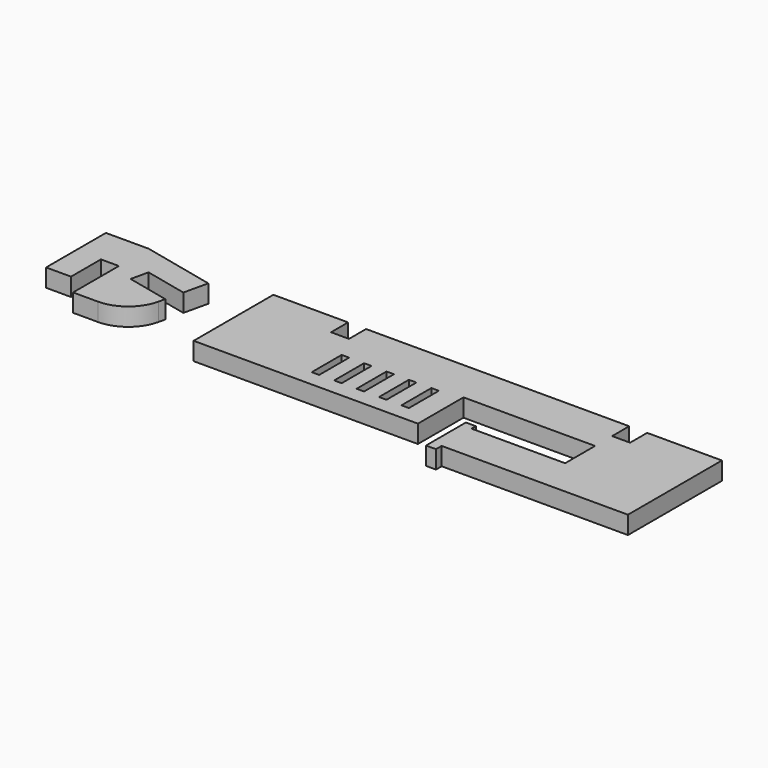
from build123d import *

# Parameters (mm, degrees)
F1_W     = 25.4
F1_H     = 38.1
F2_DEPTH = 18.288
F1_W_2   = 7.62
F1_W_3   = 95.377
F1_H_2   = 18.1300078465
F1_H_3   = 19.9699921535
F1_W_4   = 76.2


# Not quite as in the source:
# - a variable given as a bare number and used for a length is read in inches; the dataset says mm whatever the document's units were


with BuildPart() as f2:
    # F1 (on Top) → F2 (new body)
    with BuildSketch(Plane.XY):
        Polygon((-25.4, 57.9158396344), (-25.4, 19.8158396344), (-25.4, 5.8057135582), (0, 0), (37.5647200947, -8.58622066), (39.1494498942, -1.6530269181), (-4.1830109925, 8.2515343291), (-0.1079915079, 26.0797468083), (43.2244693788, 16.175185561), (48.884218663, 40.936591782), align=None)
        with BuildLine():
            Line((37.5647200947, -8.58622066), (0, 0))
            Line((0, 0), (0, -38.5335098455))
            ThreePointArc((0, -38.5335098455), (24.020555392, -30.1304546875), (37.5647200947, -8.58622066))
        make_face()
        Polygon((-69.088, 19.8158396344), (-43.688, 19.8158396344), (-25.4, 19.8158396344), (-25.4, 57.9158396344), (-69.088, 57.9158396344), align=None)
        with Locations((-56.388, 0.7658396344)):
            Rectangle(F1_W, F1_H)
        Polygon((0, 0), (-25.4, 5.8057135582), (-25.4, -38.5335098455), (0, -38.5335098455), align=None)
    extrude(amount=F2_DEPTH)


with BuildPart() as f2b:
    # F1 (on Top) → F2, piece 2 (new body)
    with BuildSketch(Plane.XY):
        Polygon((177.8, 57.9158396344), (101.6, 57.9158396344), (101.6, -43.6841603656), (330.2, -43.6841603656), (330.2, 14.3858317879), (368.935, 14.3858317879), (464.312, 14.3858317879), (464.312, -23.7141682121), (482.6, -23.7141682121), (482.6, 14.3858317879), (558.8, 14.3858317879), (558.8, 57.9158396344), (482.6, 57.9158396344), (482.6, 36.1516669545), (464.312, 36.1516669545), (464.312, 57.9158396344), (196.088, 57.9158396344), (196.088, 36.1516669545), (177.8, 36.1516669545), align=None)
        with Locations((212.598, -8.1241603656)):
            Rectangle(F1_W_2, F1_H, mode=Mode.SUBTRACT)
        with Locations((235.458, -8.1241603656)):
            Rectangle(F1_W_2, F1_H, mode=Mode.SUBTRACT)
        with Locations((258.318, -8.1241603656)):
            Rectangle(F1_W_2, F1_H, mode=Mode.SUBTRACT)
        with Locations((281.178, -8.1241603656)):
            Rectangle(F1_W_2, F1_H, mode=Mode.SUBTRACT)
        with Locations((304.038, -8.1241603656)):
            Rectangle(F1_W_2, F1_H, mode=Mode.SUBTRACT)
        Polygon((358.775, -18.2841603656), (358.775, -43.6841603656), (368.935, -43.6841603656), (368.935, -23.7141682121), (368.935, -18.2841603656), align=None)
        Polygon((368.935, -43.6841603656), (358.775, -43.6841603656), (358.775, -69.0841603656), (368.935, -69.0841603656), (368.935, -61.8141682121), align=None)
        with Locations((416.6235, -52.7491642889)):
            Rectangle(F1_W_3, F1_H_2)
        with Locations((416.6235, -33.6991642889)):
            Rectangle(F1_W_3, F1_H_3)
        Polygon((464.312, -23.7141682121), (464.312, -43.6841603656), (464.312, -61.8141682121), (558.8, -61.8141682121), (558.8, -43.6841603656), (558.8, -23.7141682121), (482.6, -23.7141682121), align=None)
        with Locations((520.7, -4.6641682121)):
            Rectangle(F1_W_4, F1_H)
    extrude(amount=F2_DEPTH)


solid = Compound([f2.part, f2b.part])
